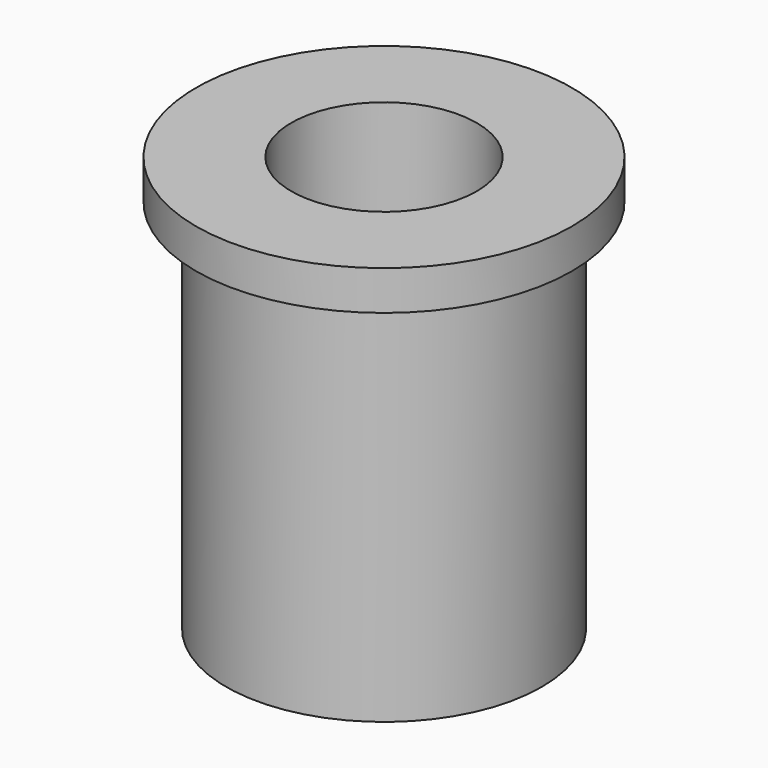
from build123d import *

# Parameters (mm, degrees)
F0_R     = 4
F0_R_2   = 2.35
F1_DEPTH = 9.525
F0_R_3   = 4.7625
F2_DEPTH = 1


# Not quite as in the source:
# - a length typed as a fraction of an inch, garbled in the dataset ("3 / 203.2 mm" for 3/8 in), is restored


with BuildPart() as f1:
    # F0 (on Top) → F1 (new body)
    with BuildSketch(Plane.XY):
        Circle(F0_R)
        Circle(F0_R_2, mode=Mode.SUBTRACT)
    extrude(amount=-F1_DEPTH)

    # F0 (on Top) → F2 (join)
    with BuildSketch(Plane.XY):
        Circle(F0_R_3)
        Circle(F0_R, mode=Mode.SUBTRACT)
        Circle(F0_R)
        Circle(F0_R_2, mode=Mode.SUBTRACT)
    extrude(amount=F2_DEPTH)


solid = f1.part
